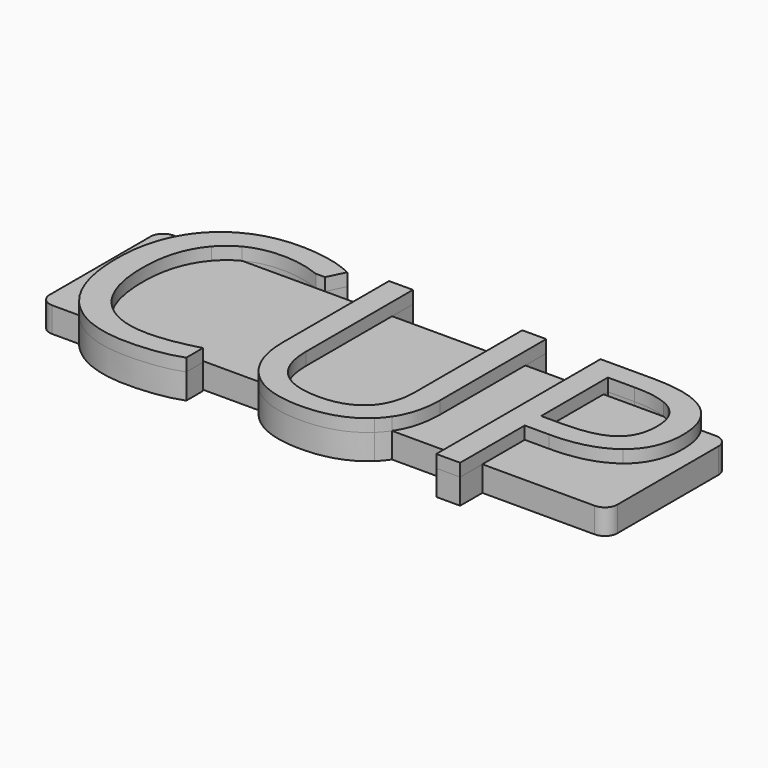
from build123d import *

# Parameters (mm, degrees)
F0_W          = 90
F0_H          = 24
F1_DEPTH      = 4
F2_R          = 2
F4_TEXT_SIZE  = 17.3611111111
F5_DEPTH      = 1.5
F3_W          = 3.7888739416
F3_H          = 4.1312020258
F3_W_2        = 3.7817519981
F3_H_2        = 4.4089578223
F6_DEPTH      = 4
F6_DEPTH_BACK = 2


# Not quite as in the source:
# - Text() gives the source's letters only with a copy of the font that has no kerning and outlines rounded to 1/6400 em; it was checked with that copy


with BuildPart() as f1:
    # F0 (on Top) → F1 (new body)
    with BuildSketch(Plane.XY):
        Rectangle(F0_W, F0_H)
    extrude(amount=F1_DEPTH)

    # F2
    f2_edges = [f1.edges().sort_by_distance(p)[0] for p in [
        (-45, -12, 2),
        (45, 12, 2),
        (-45, 12, 2),
        (45, -12, 2),
    ]]
    fillet(f2_edges, radius=F2_R)

    # F4 (on face) → F5 (cut)
    with BuildSketch(Plane(origin=(0, 0, 0), x_dir=(1, 0, 0), z_dir=(0, 0, -1))):
        with Locations((-41.3886176215, -6.25)):
            Text('16 ounces', F4_TEXT_SIZE, font='Open Sans', text_align=(TextAlign.LEFT, TextAlign.BOTTOM))
    extrude(amount=-F5_DEPTH, mode=Mode.SUBTRACT)

    # F3 (on face) → F6 (join, two sides)
    with BuildSketch(Plane.XY.offset(4)) as f6_sk:
        with BuildLine():
            add(Edge.make_bspline(
                [(-32.8065455165, -12), (-30.2694100064, -13.4960829311), (-26.6396296589, -13.4960829311)],
                knots=[0.3449081084, 0.3449081084, 0.3449081084, 1, 1, 1], degree=2))
            Line((-32.8065455165, -12), (-38.7272732331, -12))
            add(Edge.make_bspline(
                [(-38.3089340825, -12.4918888977), (-38.5240252717, -12.2515043963), (-38.7272732331, -12)],
                knots=[0, 0, 0, 0.0550614273, 0.0550614273, 0.0550614273], degree=2))
            add(Edge.make_bspline(
                [(-27.2165070824, -16.8576402627), (-34.4025480731, -16.8576402627), (-38.3089340825, -12.4918888977)],
                knots=[0, 0, 0, 1, 1, 1], degree=2))
            add(Edge.make_bspline(
                [(-18.8695893013, -15.5828123764), (-22.2525124634, -16.8576402627), (-27.2165070824, -16.8576402627)],
                knots=[0, 0, 0, 1, 1, 1], degree=2))
            Line((-18.8695893013, -15.5828123764), (-18.8695893013, -12.2711086492))
            add(Edge.make_bspline(
                [(-26.6396296589, -13.4960829311), (-23.2353406663, -13.4960829311), (-18.8695893013, -12.2711086492)],
                knots=[0, 0, 0, 1, 1, 1], degree=2))
        make_face()
        with BuildLine():
            add(Edge.make_bspline(
                [(-32.0772281246, 12), (-33.7679742448, 11.1312997435), (-35.0648888185, 9.6395505262)],
                knots=[0.5823366598, 0.5823366598, 0.5823366598, 1, 1, 1], degree=2))
            Line((-32.0772281246, 12), (-38.0979821046, 12))
            add(Edge.make_bspline(
                [(-40.335127008, 8.7172588431), (-39.4160747592, 10.5658071162), (-38.0979821046, 12)],
                knots=[0, 0, 0, 0.4888073766, 0.4888073766, 0.4888073766], degree=2))
            add(Edge.make_bspline(
                [(-42.2153200918, -0.0925852655), (-42.2153200918, 4.935506845), (-40.335127008, 8.7172588431)],
                knots=[0, 0, 0, 1, 1, 1], degree=2))
            add(Edge.make_bspline(
                [(-38.7272732331, -12), (-42.2153200918, -7.6837986785), (-42.2153200918, -0.0925852655)],
                knots=[0.0550614273, 0.0550614273, 0.0550614273, 1, 1, 1], degree=2))
            Line((-38.7272732331, -12), (-32.8065455165, -12))
            add(Edge.make_bspline(
                [(-35.1752789428, -10.0098915882), (-34.1423559894, -11.2123072498), (-32.8065455165, -12)],
                knots=[0, 0, 0, 0.3449081084, 0.3449081084, 0.3449081084], degree=2))
            add(Edge.make_bspline(
                [(-38.1700561842, -0.14243887), (-38.1700561842, -6.5237002453), (-35.1752789428, -10.0098915882)],
                knots=[0, 0, 0, 1, 1, 1], degree=2))
            add(Edge.make_bspline(
                [(-35.0648888185, 9.6395505262), (-38.1700561842, 6.0678958614), (-38.1700561842, -0.14243887)],
                knots=[0, 0, 0, 1, 1, 1], degree=2))
        make_face()
        with BuildLine():
            add(Edge.make_bspline(
                [(-26.5968979979, 13.2112051911), (-29.7198666959, 13.2112051911), (-32.0772281246, 12)],
                knots=[0, 0, 0, 0.5823366598, 0.5823366598, 0.5823366598], degree=2))
            add(Edge.make_bspline(
                [(-20.4124300873, 12), (-23.5046640426, 13.2112051911), (-26.5968979979, 13.2112051911)],
                knots=[0.1634219548, 0.1634219548, 0.1634219548, 1, 1, 1], degree=2))
            Line((-20.4124300873, 12), (-18.9480243895, 12))
            Line((-18.9480243895, 12), (-17.6018833584, 14.7281791564))
            add(Edge.make_bspline(
                [(-26.5470443934, 16.5941283532), (-21.433488961, 16.5941283532), (-17.6018833584, 14.7281791564)],
                knots=[0, 0, 0, 1, 1, 1], degree=2))
            add(Edge.make_bspline(
                [(-34.9046450898, 14.5465695972), (-31.3543562554, 16.5941283532), (-26.5470443934, 16.5941283532)],
                knots=[0, 0, 0, 1, 1, 1], degree=2))
            add(Edge.make_bspline(
                [(-38.0979821046, 12), (-36.7195265529, 13.4998726652), (-34.9046450898, 14.5465695972)],
                knots=[0.4888073766, 0.4888073766, 0.4888073766, 1, 1, 1], degree=2))
            Line((-38.0979821046, 12), (-32.0772281246, 12))
        make_face()
        with BuildLine():
            Line((-5.3215690852, -12), (-10.2277108131, -12))
            add(Edge.make_bspline(
                [(-8.8881854871, -13.6492047163), (-9.647630342, -12.8914419098), (-10.2277108131, -12)],
                knots=[0, 0, 0, 0.2361782855, 0.2361782855, 0.2361782855], degree=2))
            add(Edge.make_bspline(
                [(0.2029753897, -16.8576402627), (-5.6726279972, -16.8576402627), (-8.8881854871, -13.6492047163)],
                knots=[0, 0, 0, 1, 1, 1], degree=2))
            add(Edge.make_bspline(
                [(9.4401361083, -13.6741315186), (6.0785787766, -16.8576402627), (0.2029753897, -16.8576402627)],
                knots=[0, 0, 0, 1, 1, 1], degree=2))
            add(Edge.make_bspline(
                [(10.8659159661, -12), (10.2507667535, -12.9064368185), (9.4401361083, -13.6741315186)],
                knots=[0.7588526492, 0.7588526492, 0.7588526492, 1, 1, 1], degree=2))
            Line((10.8659159661, -12), (6.0214101004, -12))
            add(Edge.make_bspline(
                [(0.4522434122, -13.5388145921), (3.9000658378, -13.5388145921), (6.0214101004, -12)],
                knots=[0, 0, 0, 0.8375650133, 0.8375650133, 0.8375650133], degree=2))
            add(Edge.make_bspline(
                [(-5.3215690852, -12), (-3.1714362179, -13.5388145921), (0.4522434122, -13.5388145921)],
                knots=[0.1603879816, 0.1603879816, 0.1603879816, 1, 1, 1], degree=2))
        make_face()
        with BuildLine():
            Line((-8.3148690354, 12), (-12.103742977, 12))
            Line((-12.103742977, 12), (-12.103742977, -4.835799636))
            add(Edge.make_bspline(
                [(-10.2277108131, -12), (-12.103742977, -9.1169970751), (-12.103742977, -4.835799636)],
                knots=[0.2361782855, 0.2361782855, 0.2361782855, 1, 1, 1], degree=2))
            Line((-10.2277108131, -12), (-5.3215690852, -12))
            add(Edge.make_bspline(
                [(-6.0892616919, -11.3559389096), (-5.7323010223, -11.7060459343), (-5.3215690852, -12)],
                knots=[0, 0, 0, 0.1603879816, 0.1603879816, 0.1603879816], degree=2))
            add(Edge.make_bspline(
                [(-8.3148690354, -5.0993115455), (-8.3148690354, -9.173063227), (-6.0892616919, -11.3559389096)],
                knots=[0, 0, 0, 1, 1, 1], degree=2))
            Line((-8.3148690354, -5.0993115455), (-8.3148690354, 12))
        make_face()
        with BuildLine():
            Line((12.8016934399, 12), (9.0199414418, 12))
            Line((9.0199414418, 12), (9.0199414418, -5.0565798845))
            add(Edge.make_bspline(
                [(6.7943340983, -11.3452559943), (9.0199414418, -9.1516973965), (9.0199414418, -5.0565798845)],
                knots=[0, 0, 0, 1, 1, 1], degree=2))
            add(Edge.make_bspline(
                [(6.0214101004, -12), (6.4328175991, -11.7015666559), (6.7943340983, -11.3452559943)],
                knots=[0.8375650133, 0.8375650133, 0.8375650133, 1, 1, 1], degree=2))
            Line((6.0214101004, -12), (10.8659159661, -12))
            add(Edge.make_bspline(
                [(12.8016934399, -4.921262958), (12.8016934399, -9.1475864088), (10.8659159661, -12)],
                knots=[0, 0, 0, 0.7588526492, 0.7588526492, 0.7588526492], degree=2))
            Line((12.8016934399, -4.921262958), (12.8016934399, 12))
        make_face()
        with Locations((-10.2093060062, 14.0656010129)):
            Rectangle(F3_W, F3_H)
        with Locations((10.9108174408, 14.0656010129)):
            Rectangle(F3_W_2, F3_H)
        with Locations((23.3029991295, -14.2044789111)):
            Rectangle(F3_W_2, F3_H_2)
        with BuildLine():
            Line((25.1938751286, 12), (21.4121231305, 12))
            Line((21.4121231305, 12), (21.4121231305, -12))
            Line((21.4121231305, -12), (25.1938751286, -12))
            Line((25.1938751286, -12), (25.1938751286, -3.6108253541))
            Line((25.1938751286, -3.6108253541), (29.0254807312, -3.6108253541))
            add(Edge.make_bspline(
                [(38.6721532009, -0.9507794571), (35.299912954, -3.6108253541), (29.0254807312, -3.6108253541)],
                knots=[0, 0, 0, 1, 1, 1], degree=2))
            add(Edge.make_bspline(
                [(42.0443934478, 6.6518952283), (42.0443934478, 1.7092664398), (38.6721532009, -0.9507794571)],
                knots=[0, 0, 0, 1, 1, 1], degree=2))
            add(Edge.make_bspline(
                [(40.6362448919, 12), (42.0443934478, 9.8733324646), (42.0443934478, 6.6518952283)],
                knots=[0.6601610956, 0.6601610956, 0.6601610956, 1, 1, 1], degree=2))
            Line((40.6362448919, 12), (34.7323336724, 12))
            add(Edge.make_bspline(
                [(36.0121073039, 11.2775975311), (35.4542153694, 11.6936684519), (34.7323336724, 12)],
                knots=[0, 0, 0, 0.2637516041, 0.2637516041, 0.2637516041], degree=2))
            add(Edge.make_bspline(
                [(38.1273245232, 6.4738466408), (38.1273245232, 9.700087046), (36.0121073039, 11.2775975311)],
                knots=[0, 0, 0, 1, 1, 1], degree=2))
            add(Edge.make_bspline(
                [(35.8803513492, 1.2605839994), (38.1273245232, 2.8843871172), (38.1273245232, 6.4738466408)],
                knots=[0, 0, 0, 1, 1, 1], degree=2))
            add(Edge.make_bspline(
                [(28.6052860647, -0.3632191185), (33.6333781752, -0.3632191185), (35.8803513492, 1.2605839994)],
                knots=[0, 0, 0, 1, 1, 1], degree=2))
            Line((28.6052860647, -0.3632191185), (25.1938751286, -0.3632191185))
            Line((25.1938751286, -0.3632191185), (25.1938751286, 12))
        make_face()
        with BuildLine():
            Line((21.4121231305, 16.1312020258), (21.4121231305, 12))
            Line((21.4121231305, 12), (25.1938751286, 12))
            Line((25.1938751286, 12), (25.1938751286, 12.8551080161))
            Line((25.1938751286, 12.8551080161), (29.4243095671, 12.8551080161))
            add(Edge.make_bspline(
                [(34.7323336724, 12), (32.7172397989, 12.8551080161), (29.4243095671, 12.8551080161)],
                knots=[0.2637516041, 0.2637516041, 0.2637516041, 1, 1, 1], degree=2))
            Line((34.7323336724, 12), (40.6362448919, 12))
            add(Edge.make_bspline(
                [(29.8516261771, 16.1312020258), (37.9008167772, 16.1312020258), (40.6362448919, 12)],
                knots=[0, 0, 0, 0.6601610956, 0.6601610956, 0.6601610956], degree=2))
            Line((29.8516261771, 16.1312020258), (21.4121231305, 16.1312020258))
        make_face()
    extrude(amount=-F6_DEPTH)
    extrude(f6_sk.sketch, amount=F6_DEPTH_BACK)


solid = f1.part
